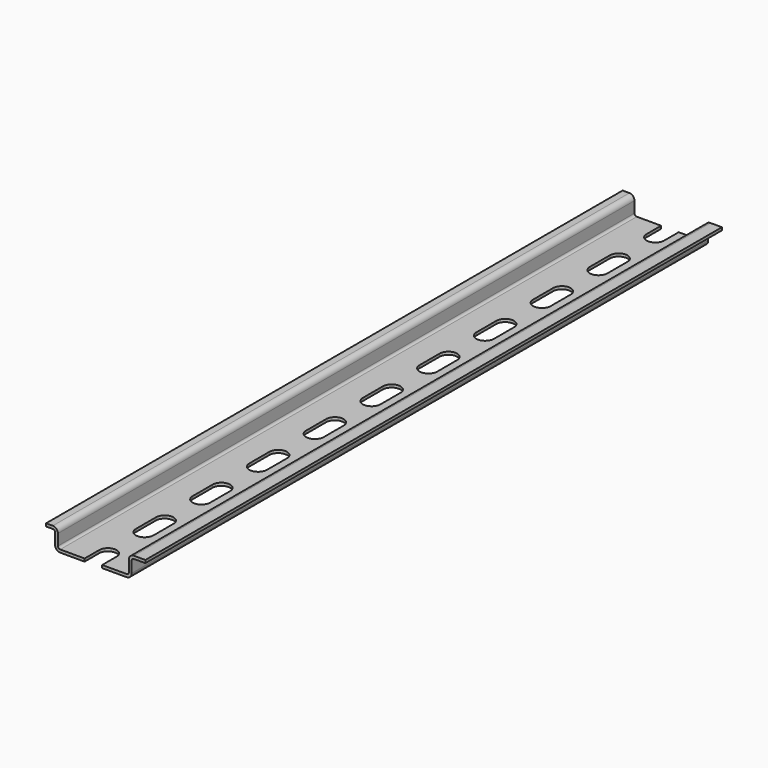
from build123d import *

# Parameters (mm, degrees)
F1_DEPTH = 127
F3_DEPTH = 1.001
F4_DEPTH = 1


# Not quite as in the source:
# - a feature names something its author has since deleted; it is built from what else it names


with BuildPart() as f1:
    # F0 (on Front) → F1 (new body, symmetric)
    with BuildSketch(Plane.XZ):
        with BuildLine():
            ThreePointArc((-13.5001, 1.8), (-12.9728922061, 0.5272077939), (-11.7001, 0))
            Line((-11.7001, 0), (11.7001, 0))
            ThreePointArc((11.7001, 0), (12.9728922061, 0.5272077939), (13.5001, 1.8))
            Line((13.5001, 1.8), (13.5001, 5.70062))
            ThreePointArc((13.5001, 5.70062), (13.7344145751, 6.2663054249), (14.3001, 6.50062))
            Line((14.3001, 6.50062), (18.3269093243, 6.50062))
            Line((18.3269093243, 6.50062), (18.3269093243, 7.50062))
            Line((18.3269093243, 7.50062), (14.2999, 7.50062))
            ThreePointArc((14.2999, 7.50062), (13.0271077939, 6.9734122061), (12.4999, 5.70062))
            Line((12.4999, 5.70062), (12.4999, 1.8))
            ThreePointArc((12.4999, 1.8), (12.2655854249, 1.2343145751), (11.6999, 1))
            Line((11.6999, 1), (-11.7001, 1))
            ThreePointArc((-11.7001, 1), (-12.2657854249, 1.2343145751), (-12.5001, 1.8))
            Line((-12.5001, 1.8), (-12.5001, 5.70062))
            ThreePointArc((-12.5001, 5.70062), (-13.0273077939, 6.9734122061), (-14.3001, 7.50062))
            Line((-14.3001, 7.50062), (-16.6730906757, 7.50062))
            Line((-16.6730906757, 7.50062), (-16.6730906757, 6.50062))
            Line((-16.6730906757, 6.50062), (-14.3001, 6.50062))
            ThreePointArc((-14.3001, 6.50062), (-13.7344145751, 6.2663054249), (-13.5001, 5.70062))
            Line((-13.5001, 5.70062), (-13.5001, 1.8))
        make_face()
    extrude(amount=F1_DEPTH, both=True)

    # F2 (on face) → F3 (cut, through all)
    with BuildSketch(Plane.XY.offset(1)):
        with BuildLine():
            ThreePointArc((-3.1, -4.4), (0, -7.5), (3.1, -4.4))
            Line((3.1, -4.4), (3.1, 4.4))
            ThreePointArc((3.1, 4.4), (0, 7.5), (-3.1, 4.4))
            Line((-3.1, 4.4), (-3.1, -4.4))
        make_face()
        with BuildLine():
            ThreePointArc((-3.1, 20.6), (0, 17.5), (3.1, 20.6))
            Line((3.1, 20.6), (3.1, 29.4))
            ThreePointArc((3.1, 29.4), (0, 32.5), (-3.1, 29.4))
            Line((-3.1, 29.4), (-3.1, 20.6))
        make_face()
        with BuildLine():
            ThreePointArc((-3.1, 45.6), (0, 42.5), (3.1, 45.6))
            Line((3.1, 45.6), (3.1, 54.4))
            ThreePointArc((3.1, 54.4), (0, 57.5), (-3.1, 54.4))
            Line((-3.1, 54.4), (-3.1, 45.6))
        make_face()
        with BuildLine():
            ThreePointArc((-3.1, 70.6), (0, 67.5), (3.1, 70.6))
            Line((3.1, 70.6), (3.1, 79.4))
            ThreePointArc((3.1, 79.4), (0, 82.5), (-3.1, 79.4))
            Line((-3.1, 79.4), (-3.1, 70.6))
        make_face()
        with BuildLine():
            ThreePointArc((-3.1, 95.6), (0, 92.5), (3.1, 95.6))
            Line((3.1, 95.6), (3.1, 104.4))
            ThreePointArc((3.1, 104.4), (0, 107.5), (-3.1, 104.4))
            Line((-3.1, 104.4), (-3.1, 95.6))
        make_face()
        with BuildLine():
            ThreePointArc((-3.1, 120.6), (0, 117.5), (3.1, 120.6))
            Line((3.1, 120.6), (3.1, 129.4))
            ThreePointArc((3.1, 129.4), (0, 132.5), (-3.1, 129.4))
            Line((-3.1, 129.4), (-3.1, 120.6))
        make_face()
        with BuildLine():
            ThreePointArc((-3.1, -29.4), (0, -32.5), (3.1, -29.4))
            Line((3.1, -29.4), (3.1, -20.6))
            ThreePointArc((3.1, -20.6), (0, -17.5), (-3.1, -20.6))
            Line((-3.1, -20.6), (-3.1, -29.4))
        make_face()
        with BuildLine():
            ThreePointArc((3.1, -45.6), (0, -42.5), (-3.1, -45.6))
            Line((-3.1, -45.6), (-3.1, -54.4))
            ThreePointArc((-3.1, -54.4), (0, -57.5), (3.1, -54.4))
            Line((3.1, -54.4), (3.1, -45.6))
        make_face()
        with BuildLine():
            ThreePointArc((-3.1, -79.4), (0, -82.5), (3.1, -79.4))
            Line((3.1, -79.4), (3.1, -70.6))
            ThreePointArc((3.1, -70.6), (0, -67.5), (-3.1, -70.6))
            Line((-3.1, -70.6), (-3.1, -79.4))
        make_face()
        with BuildLine():
            ThreePointArc((3.1, -95.6), (0, -92.5), (-3.1, -95.6))
            Line((-3.1, -95.6), (-3.1, -104.4))
            ThreePointArc((-3.1, -104.4), (0, -107.5), (3.1, -104.4))
            Line((3.1, -104.4), (3.1, -95.6))
        make_face()
        with BuildLine():
            ThreePointArc((3.1, -120.6), (0, -117.5), (-3.1, -120.6))
            Line((-3.1, -120.6), (-3.1, -129.4))
            ThreePointArc((-3.1, -129.4), (0, -132.5), (3.1, -129.4))
            Line((3.1, -129.4), (3.1, -120.6))
        make_face()
    extrude(amount=-F3_DEPTH, mode=Mode.SUBTRACT)

    # F2 (on face) → F4 (cut, through all)
    with BuildSketch(Plane.XY.offset(1)):
        with BuildLine():
            ThreePointArc((-3.1, 95.6), (0, 92.5), (3.1, 95.6))
            Line((3.1, 95.6), (3.1, 104.4))
            ThreePointArc((3.1, 104.4), (0, 107.5), (-3.1, 104.4))
            Line((-3.1, 104.4), (-3.1, 95.6))
        make_face()
        with BuildLine():
            ThreePointArc((-3.1, 70.6), (0, 67.5), (3.1, 70.6))
            Line((3.1, 70.6), (3.1, 79.4))
            ThreePointArc((3.1, 79.4), (0, 82.5), (-3.1, 79.4))
            Line((-3.1, 79.4), (-3.1, 70.6))
        make_face()
        with BuildLine():
            ThreePointArc((-3.1, 45.6), (0, 42.5), (3.1, 45.6))
            Line((3.1, 45.6), (3.1, 54.4))
            ThreePointArc((3.1, 54.4), (0, 57.5), (-3.1, 54.4))
            Line((-3.1, 54.4), (-3.1, 45.6))
        make_face()
        with BuildLine():
            ThreePointArc((-3.1, 20.6), (0, 17.5), (3.1, 20.6))
            Line((3.1, 20.6), (3.1, 29.4))
            ThreePointArc((3.1, 29.4), (0, 32.5), (-3.1, 29.4))
            Line((-3.1, 29.4), (-3.1, 20.6))
        make_face()
        with BuildLine():
            ThreePointArc((-3.1, -4.4), (0, -7.5), (3.1, -4.4))
            Line((3.1, -4.4), (3.1, 4.4))
            ThreePointArc((3.1, 4.4), (0, 7.5), (-3.1, 4.4))
            Line((-3.1, 4.4), (-3.1, -4.4))
        make_face()
        with BuildLine():
            ThreePointArc((-3.1, 120.6), (0, 117.5), (3.1, 120.6))
            Line((3.1, 120.6), (3.1, 127))
            Line((3.1, 127), (-3.1, 127))
            Line((-3.1, 127), (-3.1, 120.6))
        make_face()
        with BuildLine():
            Line((-3.1, 127), (3.1, 127))
            Line((3.1, 127), (3.1, 129.4))
            ThreePointArc((3.1, 129.4), (0, 132.5), (-3.1, 129.4))
            Line((-3.1, 129.4), (-3.1, 127))
        make_face()
    extrude(amount=-F4_DEPTH, mode=Mode.SUBTRACT)


solid = f1.part
